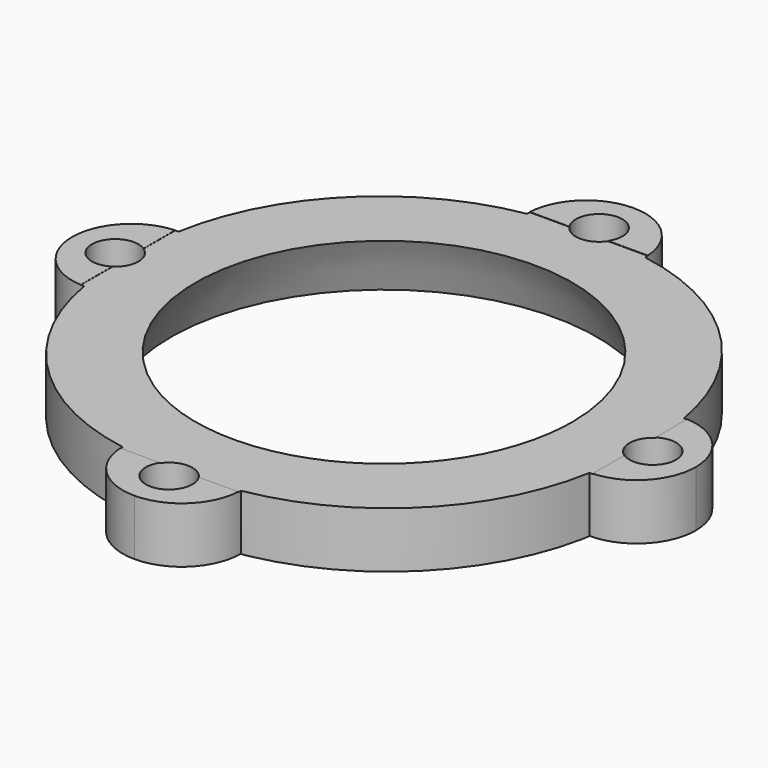
from build123d import *

# Parameters (mm, degrees)
F3_W          = 55
F3_H          = 55
F4_DEPTH      = 6
F7_W          = 12.7
F7_H          = 6
F8_DEPTH      = 6
F10_W         = 12.7
F10_H         = 6
F11_DEPTH     = 6
F13_W         = 12.7
F13_H         = 6
F14_DEPTH     = 6
F16_W         = 12.7
F16_H         = 6
F17_DEPTH     = 6
F19_D         = 5
F21_D         = 5
F23_D         = 5
F25_D         = 5
F26_T4_DEPTH  = 133
F26_T10_DEPTH = 133
F26_T15_DEPTH = 133
F26_T21_DEPTH = 133
F26_T27_DEPTH = 133
F26_T33_DEPTH = 133
F26_T38_DEPTH = 133
F26_T44_DEPTH = 133
F26_T49_DEPTH = 133
F26_T55_DEPTH = 133
F26_T61_DEPTH = 133
F26_T66_DEPTH = 133
F27_R         = 6.34999


# Not quite as in the source:
# - a fillet or chamfer that OpenCascade refuses, or shapes differently, is made with other operations: its cross-section is extruded or revolved along the edge and cut away or added
# - a fillet or chamfer is up to 0.001 mm smaller than in the source, because OpenCascade refuses the exact size


with BuildPart() as f1:
    # F0 (on Front) → F1 (revolve)
    with BuildSketch(Plane.XZ):
        with BuildLine():
            Line((0, 0), (0, -32.5))
            add(Edge.make_bspline(
                [(0, -32.5), (25, -32.5), (25, 0)],
                knots=[0, 0, 0, 1.5707963268, 1.5707963268, 1.5707963268], degree=2, weights=[1, 0.7071067812, 1]))
            Line((25, 0), (0, 0))
        make_face()
        with BuildLine():
            Line((0, 0), (25, 0))
            add(Edge.make_bspline(
                [(25, 0), (25, 32.5), (0, 32.5)],
                knots=[1.5707963268, 1.5707963268, 1.5707963268, 3.1415926536, 3.1415926536, 3.1415926536], degree=2, weights=[1, 0.7071067812, 1]))
            Line((0, 32.5), (0, 0))
        make_face()
    revolve(axis=Axis((0, 0, 0), (0, 0, -1)))


with BuildPart() as f4:
    # F3 (on offset) → F4 (new body)
    with BuildSketch(Plane.XY.offset(19.05)):
        Rectangle(F3_W, F3_H)
    extrude(amount=-F4_DEPTH)

    # F5: cut F1
    add(f1.part, mode=Mode.SUBTRACT)

    # F7 (on offset) → F8 (join)
    with BuildSketch(Plane.XZ.offset(27.5)):
        with Locations((0, 16.0963926464)):
            Rectangle(F7_W, F7_H)
    extrude(amount=F8_DEPTH)

    # F10 (on offset) → F11 (join)
    with BuildSketch(Plane.YZ.offset(27.5)):
        with Locations((0, 16.087366268)):
            Rectangle(F10_W, F10_H)
    extrude(amount=F11_DEPTH)

    # F13 (on offset) → F14 (join)
    with BuildSketch(Plane.XZ.offset(-27.5)):
        with Locations((0, 16.07888937)):
            Rectangle(F13_W, F13_H)
    extrude(amount=-F14_DEPTH)

    # F16 (on offset) → F17 (join)
    with BuildSketch(Plane.YZ.offset(-27.5)):
        with Locations((0, 16.0636380315)):
            Rectangle(F16_W, F16_H)
    extrude(amount=-F17_DEPTH)

    # F19 (through all)
    with Locations(Plane.XY.offset(19.07888937)):
        with Locations((0, 28.8921689615)):
            Hole(F19_D / 2)

    # F21 (through all)
    with Locations(Plane.XY.offset(19.0636380315)):
        with Locations((-28.8809893653, 0)):
            Hole(F21_D / 2)

    # F23 (through all)
    with Locations(Plane.XY.offset(19.087366268)):
        with Locations((28.8808012381, 0)):
            Hole(F23_D / 2)

    # F25 (through all)
    with Locations(Plane.XY.offset(19.0963926464)):
        with Locations((0, -28.8607433438)):
            Hole(F25_D / 2)

    # F26: fillet of radius 25.4 on 4 edges, made by hand


with BuildPart() as f26_tool2:
    # F26_s3 → F26_t4 (new body)
    with BuildSketch(Plane.XY.offset(82.55)):
        with BuildLine():
            ThreePointArc((-27.5, 2.1), (-20.0605122421, 20.0605122421), (-2.1, 27.5))
            Line((-2.1, 27.5), (-27.5, 27.5))
            Line((-27.5, 27.5), (-27.5, 2.1))
        make_face()
    extrude(amount=-F26_T4_DEPTH)

    split(bisect_by=Plane.XZ.offset(-6.35), keep=Keep.BOTTOM)

    split(bisect_by=Plane.YZ.offset(-6.35), keep=Keep.BOTTOM)


with BuildPart() as f4_1:
    add(f4.part)

    # F26_t1: cut F26_tool2
    add(f26_tool2.part, mode=Mode.SUBTRACT)


with BuildPart() as f26_tool8:
    # F26_s9 → F26_t10 (new body)
    with BuildSketch(Plane.XY.offset(82.55)):
        with BuildLine():
            ThreePointArc((-27.5, 2.1), (-20.0605122421, 20.0605122421), (-2.1, 27.5))
            Line((-2.1, 27.5), (-27.5, 27.5))
            Line((-27.5, 27.5), (-27.5, 2.1))
        make_face()
    extrude(amount=-F26_T10_DEPTH)

    split(bisect_by=Plane.XY.offset(13.0636380315), keep=Keep.BOTTOM)


with BuildPart() as f4_2:
    add(f4_1.part)

    # F26_t7: cut F26_tool8
    add(f26_tool8.part, mode=Mode.SUBTRACT)


with BuildPart() as f26_tool13:
    # F26_s14 → F26_t15 (new body)
    with BuildSketch(Plane.XY.offset(82.55)):
        with BuildLine():
            ThreePointArc((-27.5, 2.1), (-20.0605122421, 20.0605122421), (-2.1, 27.5))
            Line((-2.1, 27.5), (-27.5, 27.5))
            Line((-27.5, 27.5), (-27.5, 2.1))
        make_face()
    extrude(amount=-F26_T15_DEPTH)

    split(bisect_by=Plane.XY.offset(13.07888937), keep=Keep.BOTTOM)

    split(bisect_by=Plane.YZ.offset(-6.35), keep=Keep.TOP)


with BuildPart() as f4_3:
    add(f4_2.part)

    # F26_t12: cut F26_tool13
    add(f26_tool13.part, mode=Mode.SUBTRACT)


with BuildPart() as f26_tool19:
    # F26_s20 → F26_t21 (new body)
    with BuildSketch(Plane.XY.offset(82.55)):
        with BuildLine():
            ThreePointArc((-2.1, -27.5), (-20.0605122421, -20.0605122421), (-27.5, -2.1))
            Line((-27.5, -2.1), (-27.5, -27.5))
            Line((-27.5, -27.5), (-2.1, -27.5))
        make_face()
    extrude(amount=-F26_T21_DEPTH)

    split(bisect_by=Plane.YZ.offset(-6.35), keep=Keep.BOTTOM)

    split(bisect_by=Plane.XZ.offset(6.35), keep=Keep.TOP)


with BuildPart() as f4_4:
    add(f4_3.part)

    # F26_t18: cut F26_tool19
    add(f26_tool19.part, mode=Mode.SUBTRACT)


with BuildPart() as f26_tool25:
    # F26_s26 → F26_t27 (new body)
    with BuildSketch(Plane.XY.offset(82.55)):
        with BuildLine():
            ThreePointArc((-2.1, -27.5), (-20.0605122421, -20.0605122421), (-27.5, -2.1))
            Line((-27.5, -2.1), (-27.5, -27.5))
            Line((-27.5, -27.5), (-2.1, -27.5))
        make_face()
    extrude(amount=-F26_T27_DEPTH)

    split(bisect_by=Plane.XY.offset(13.0963926464), keep=Keep.BOTTOM)

    split(bisect_by=Plane.XZ.offset(6.35), keep=Keep.TOP)


with BuildPart() as f4_5:
    add(f4_4.part)

    # F26_t24: cut F26_tool25
    add(f26_tool25.part, mode=Mode.SUBTRACT)


with BuildPart() as f26_tool31:
    # F26_s32 → F26_t33 (new body)
    with BuildSketch(Plane.XY.offset(82.55)):
        with BuildLine():
            ThreePointArc((-2.1, -27.5), (-20.0605122421, -20.0605122421), (-27.5, -2.1))
            Line((-27.5, -2.1), (-27.5, -27.5))
            Line((-27.5, -27.5), (-2.1, -27.5))
        make_face()
    extrude(amount=-F26_T33_DEPTH)

    split(bisect_by=Plane.XY.offset(13.0636380315), keep=Keep.BOTTOM)


with BuildPart() as f4_6:
    add(f4_5.part)

    # F26_t30: cut F26_tool31
    add(f26_tool31.part, mode=Mode.SUBTRACT)


with BuildPart() as f26_tool36:
    # F26_s37 → F26_t38 (new body)
    with BuildSketch(Plane.XY.offset(82.55)):
        with BuildLine():
            ThreePointArc((27.5, -2.1), (20.0605122421, -20.0605122421), (2.1, -27.5))
            Line((2.1, -27.5), (27.5, -27.5))
            Line((27.5, -27.5), (27.5, -2.1))
        make_face()
    extrude(amount=-F26_T38_DEPTH)

    split(bisect_by=Plane.YZ.offset(6.35), keep=Keep.TOP)

    split(bisect_by=Plane.XZ.offset(6.35), keep=Keep.TOP)


with BuildPart() as f4_7:
    add(f4_6.part)

    # F26_t35: cut F26_tool36
    add(f26_tool36.part, mode=Mode.SUBTRACT)


with BuildPart() as f26_tool42:
    # F26_s43 → F26_t44 (new body)
    with BuildSketch(Plane.XY.offset(82.55)):
        with BuildLine():
            ThreePointArc((27.5, -2.1), (20.0605122421, -20.0605122421), (2.1, -27.5))
            Line((2.1, -27.5), (27.5, -27.5))
            Line((27.5, -27.5), (27.5, -2.1))
        make_face()
    extrude(amount=-F26_T44_DEPTH)

    split(bisect_by=Plane.XY.offset(13.087366268), keep=Keep.BOTTOM)


with BuildPart() as f4_8:
    add(f4_7.part)

    # F26_t41: cut F26_tool42
    add(f26_tool42.part, mode=Mode.SUBTRACT)


with BuildPart() as f26_tool47:
    # F26_s48 → F26_t49 (new body)
    with BuildSketch(Plane.XY.offset(82.55)):
        with BuildLine():
            ThreePointArc((27.5, -2.1), (20.0605122421, -20.0605122421), (2.1, -27.5))
            Line((2.1, -27.5), (27.5, -27.5))
            Line((27.5, -27.5), (27.5, -2.1))
        make_face()
    extrude(amount=-F26_T49_DEPTH)

    split(bisect_by=Plane.XY.offset(13.0963926464), keep=Keep.BOTTOM)

    split(bisect_by=Plane.XZ.offset(6.35), keep=Keep.TOP)


with BuildPart() as f4_9:
    add(f4_8.part)

    # F26_t46: cut F26_tool47
    add(f26_tool47.part, mode=Mode.SUBTRACT)


with BuildPart() as f26_tool53:
    # F26_s54 → F26_t55 (new body)
    with BuildSketch(Plane.XY.offset(82.55)):
        with BuildLine():
            ThreePointArc((2.1, 27.5), (20.0605122421, 20.0605122421), (27.5, 2.1))
            Line((27.5, 2.1), (27.5, 27.5))
            Line((27.5, 27.5), (2.1, 27.5))
        make_face()
    extrude(amount=-F26_T55_DEPTH)

    split(bisect_by=Plane.YZ.offset(6.35), keep=Keep.TOP)

    split(bisect_by=Plane.XZ.offset(-6.35), keep=Keep.BOTTOM)


with BuildPart() as f4_10:
    add(f4_9.part)

    # F26_t52: cut F26_tool53
    add(f26_tool53.part, mode=Mode.SUBTRACT)


with BuildPart() as f26_tool59:
    # F26_s60 → F26_t61 (new body)
    with BuildSketch(Plane.XY.offset(82.55)):
        with BuildLine():
            ThreePointArc((2.1, 27.5), (20.0605122421, 20.0605122421), (27.5, 2.1))
            Line((27.5, 2.1), (27.5, 27.5))
            Line((27.5, 27.5), (2.1, 27.5))
        make_face()
    extrude(amount=-F26_T61_DEPTH)

    split(bisect_by=Plane.XY.offset(13.07888937), keep=Keep.BOTTOM)


with BuildPart() as f4_11:
    add(f4_10.part)

    # F26_t58: cut F26_tool59
    add(f26_tool59.part, mode=Mode.SUBTRACT)


with BuildPart() as f26_tool64:
    # F26_s65 → F26_t66 (new body)
    with BuildSketch(Plane.XY.offset(82.55)):
        with BuildLine():
            ThreePointArc((2.1, 27.5), (20.0605122421, 20.0605122421), (27.5, 2.1))
            Line((27.5, 2.1), (27.5, 27.5))
            Line((27.5, 27.5), (2.1, 27.5))
        make_face()
    extrude(amount=-F26_T66_DEPTH)

    split(bisect_by=Plane.XY.offset(13.087366268), keep=Keep.BOTTOM)

    split(bisect_by=Plane.XZ.offset(-6.35), keep=Keep.TOP)


with BuildPart() as f4_12:
    add(f4_11.part)

    # F26_t63: cut F26_tool64
    add(f26_tool64.part, mode=Mode.SUBTRACT)

    # F27 (radius 6.35 in the source; OpenCascade refuses exactly that, so slightly less here)
    f27_edges = [f4_12.edges().sort_by_distance(p)[0] for p in [
        (6.35, 33.5, 16.078889),
        (-6.35, 33.5, 16.078889),
        (-33.5, 6.35, 16.063638),
        (-33.5, -6.35, 16.063638),
        (-6.35, -33.5, 16.096393),
        (6.35, -33.5, 16.096393),
        (33.5, -6.35, 16.087366),
        (33.5, 6.35, 16.087366),
    ]]
    fillet(f27_edges, radius=F27_R)


solid = f4_12.part
